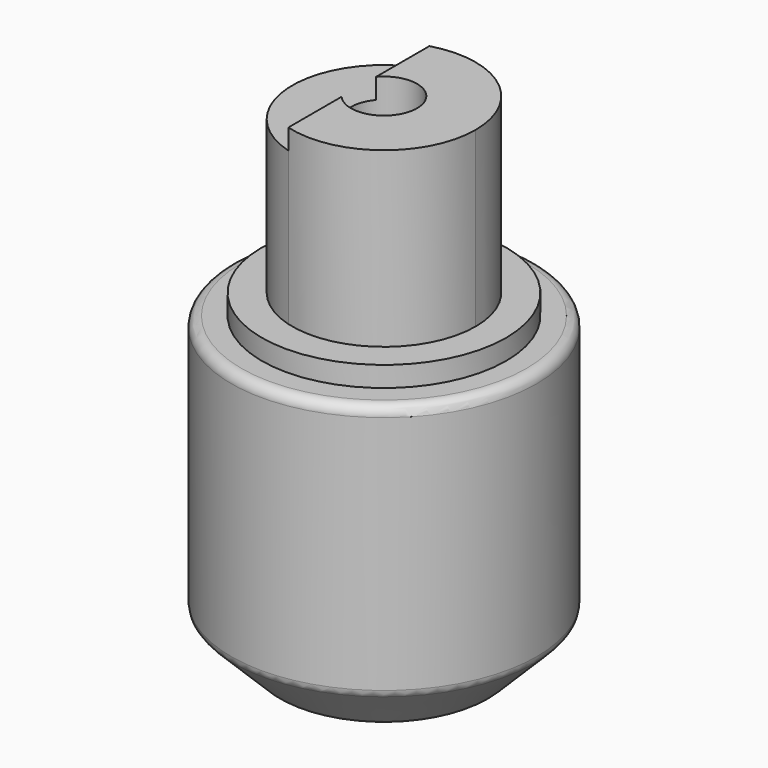
from build123d import *

# Parameters (mm, degrees)
F0_R           = 15
F1_DEPTH       = 30
F2_R           = 12
F3_DEPTH       = 2
F5_DEPTH       = 17
F6_DEPTH       = 15
F7_D           = 6.5
F7_CBORE_D     = 13
F7_CBORE_DEPTH = 15
F8_SIZE        = 5
F9_R           = 1


with BuildPart() as f1:
    # F0 (on Top) → F1 (new body)
    with BuildSketch(Plane.XY):
        Circle(F0_R)
    extrude(amount=F1_DEPTH)

    # F2 (on face) → F3 (join)
    with BuildSketch(Plane.XY.offset(30)):
        Circle(F2_R)
    extrude(amount=F3_DEPTH)

    # F4 (on face) → F5 (join)
    with BuildSketch(Plane.XY.offset(32)):
        with BuildLine():
            ThreePointArc((-2.4664324925, -8.6554439955), (5.4222738573, -7.1832406486), (9, 0))
            ThreePointArc((9, 0), (5.4222738573, 7.1832406486), (-2.4664324925, 8.6554439955))
            Line((-2.4664324925, 8.6554439955), (-2.4664324925, -8.6554439955))
        make_face()
    extrude(amount=F5_DEPTH)

    # F4 (on face) → F6 (join)
    with BuildSketch(Plane.XY.offset(32)):
        with BuildLine():
            Line((-2.4664324925, -8.6554439955), (-2.4664324925, 8.6554439955))
            ThreePointArc((-2.4664324925, 8.6554439955), (-9, 0), (-2.4664324925, -8.6554439955))
        make_face()
    extrude(amount=F6_DEPTH)

    # F7 (through all)
    with Locations(Plane(origin=(0, 0, 0), x_dir=(1, 0, 0), z_dir=(0, 0, -1))):
        with Locations((0, 0)):
            CounterBoreHole(F7_D / 2, F7_CBORE_D / 2, F7_CBORE_DEPTH)

    # F8
    f8_edges = [f1.edges().sort_by_distance(p)[0] for p in [
        (-15, 0, 0),
    ]]
    chamfer(f8_edges, length=F8_SIZE)

    # F9
    f9_edges = [f1.edges().sort_by_distance(p)[0] for p in [
        (-15, 0, 30),
        (-10, 0, 0),
        (-15, 0, 5),
        (-6.5, 0, 0),
    ]]
    fillet(f9_edges, radius=F9_R)


solid = f1.part
